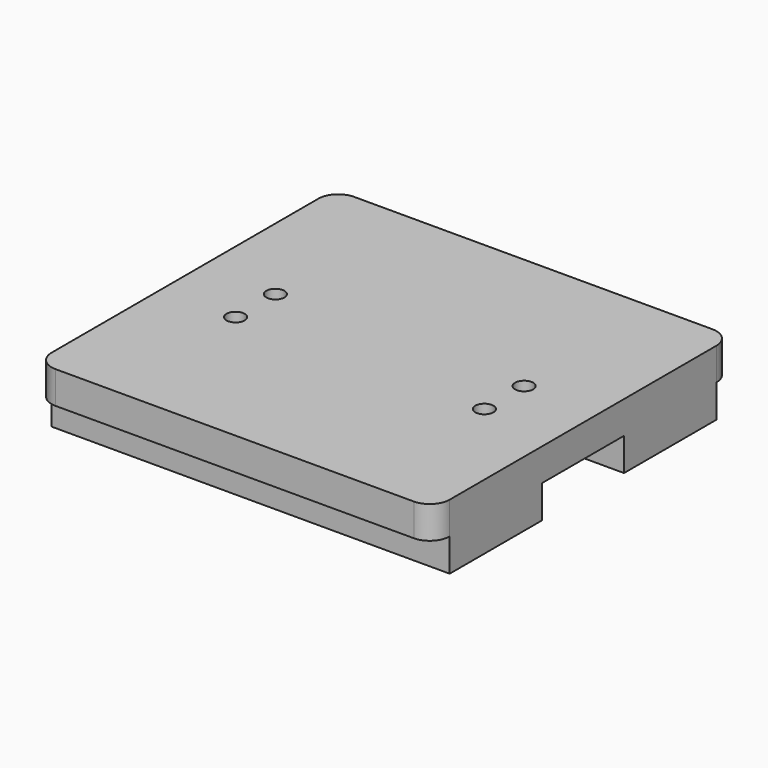
from build123d import *

# Parameters (mm, degrees)
F0_W     = 101.6
F0_H     = 95.25
F0_R     = 2.3114
F1_DEPTH = 8.255
F2_R     = 5.08
F3_W     = 101.6
F3_H     = 29.464
F4_DEPTH = 8.382


# Not quite as in the source:
# - a feature names something its author has since deleted; it is built from what else it names


with BuildPart() as f1:
    # F0 (on Top) → F1 (new body)
    with BuildSketch(Plane.XY):
        Rectangle(F0_W, F0_H)
        Polygon((38.1, -15.24), (0, -15.24), (-38.1, -15.24), (-38.1, 15.24), (-25.4, 15.24), (0, 15.24), (25.4, 15.24), (38.1, 15.24), align=None, mode=Mode.SUBTRACT)
        Polygon((-38.1, -15.24), (0, -15.24), (38.1, -15.24), (38.1, 15.24), (25.4, 15.24), (0, 15.24), (-25.4, 15.24), (-38.1, 15.24), align=None)
        with Locations((-31.75, -7.6708)):
            Circle(F0_R, mode=Mode.SUBTRACT)
        with Locations((31.75, -7.6708)):
            Circle(F0_R, mode=Mode.SUBTRACT)
        with Locations((-31.75, 5.0292)):
            Circle(F0_R, mode=Mode.SUBTRACT)
        with Locations((31.75, 5.0292)):
            Circle(F0_R, mode=Mode.SUBTRACT)
    extrude(amount=F1_DEPTH)

    # F2
    f2_edges = [f1.edges().sort_by_distance(p)[0] for p in [
        (-50.8, 47.625, 4.1275),
        (50.8, 47.625, 4.1275),
        (50.8, -47.625, 4.1275),
        (-50.8, -47.625, 4.1275),
    ]]
    fillet(f2_edges, radius=F2_R)

    # F3 (on face) → F4 (join)
    with BuildSketch(Plane(origin=(0, 0, 0), x_dir=(1, 0, 0), z_dir=(0, 0, -1))):
        with Locations((0, 27.813)):
            Rectangle(F3_W, F3_H)
        with Locations((0, -27.813)):
            Rectangle(F3_W, F3_H)
    extrude(amount=F4_DEPTH)


solid = f1.part
